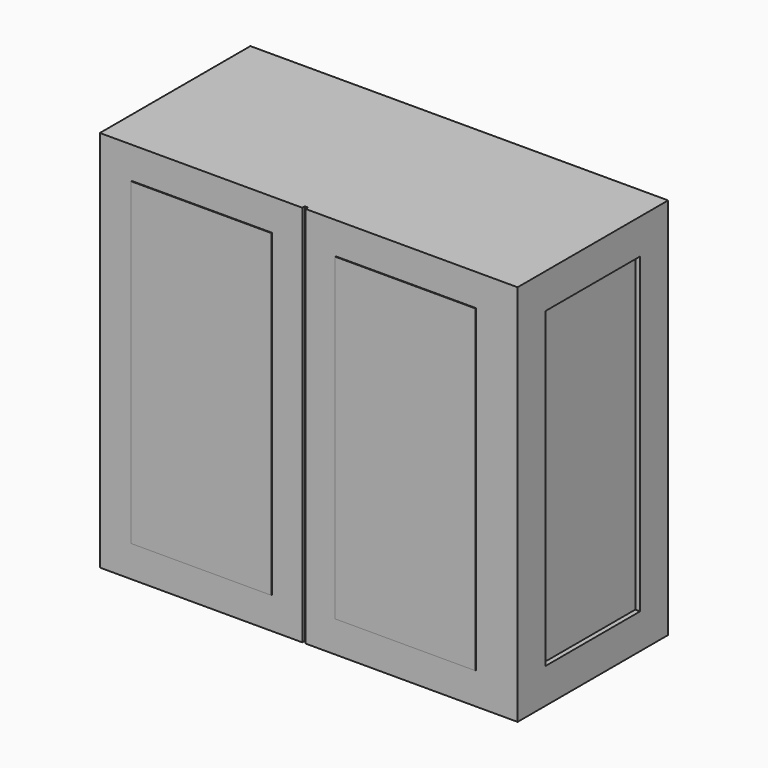
from build123d import *

# Parameters (mm, degrees)
F0_W     = 279.4
F0_H     = 635
F0_W_2   = 3.175
F0_H_2   = 762
F1_DEPTH = 374.65
F2_DEPTH = 6.35
F3_DEPTH = 1.524
F4_W     = 374.65
F4_H     = 762
F4_W_2   = 234.95
F4_H_2   = 622.3
F5_DEPTH = 19.05
F6_DEPTH = 9.525


# Not quite as in the source:
# - a feature names something its author has since deleted; it is built from what else it names


with BuildPart() as f1:
    # F0 (on Front) → F1 (new body)
    with BuildSketch(Plane.XZ):
        Polygon((-178.4927574873, 0), (224.7322425127, 0), (224.7322425127, 762), (151.7072425127, 762), (-178.4927574873, 762), align=None)
        with Locations((24.7072425127, 381)):
            Rectangle(F0_W, F0_H, mode=Mode.SUBTRACT)
        Polygon((231.0822425127, 762), (231.0822425127, 0), (634.3072425127, 0), (634.3072425127, 762), (304.1072425127, 762), align=None)
        with Locations((431.1072425127, 381)):
            Rectangle(F0_W, F0_H, mode=Mode.SUBTRACT)
        with Locations((24.7072425127, 381)):
            Rectangle(F0_W, F0_H)
        with Locations((431.1072425127, 381)):
            Rectangle(F0_W, F0_H)
        with Locations((226.3197425127, 381)):
            Rectangle(F0_W_2, F0_H_2)
        with Locations((229.4947425127, 381)):
            Rectangle(F0_W_2, F0_H_2)
    extrude(amount=-F1_DEPTH)

    # F0 (on Front) → F2 (cut)
    with BuildSketch(Plane.XZ):
        with Locations((226.3197425127, 381)):
            Rectangle(F0_W_2, F0_H_2)
        with Locations((229.4947425127, 381)):
            Rectangle(F0_W_2, F0_H_2)
        with Locations((24.7072425127, 381)):
            Rectangle(F0_W, F0_H)
        with Locations((431.1072425127, 381)):
            Rectangle(F0_W, F0_H)
    extrude(amount=-F2_DEPTH, mode=Mode.SUBTRACT)

    # F4 (on face) → F5 (join)
    with BuildSketch(Plane.YZ.offset(634.3072425127)):
        with Locations((187.325, 381)):
            Rectangle(F4_W, F4_H)
        with Locations((187.325, 381)):
            Rectangle(F4_W_2, F4_H_2, mode=Mode.SUBTRACT)
    extrude(amount=F5_DEPTH)

    # F6 (add): a face of the model
    f6_faces = [f1.faces().sort_by_distance(p)[0] for p in [
        (634.3072425127, 187.325, 381),
    ]]
    extrude(f6_faces, amount=F6_DEPTH)


with BuildPart() as f3:
    # F0 (on Front) → F3 (new body)
    with BuildSketch(Plane.XZ):
        with Locations((24.7072425127, 381)):
            Rectangle(F0_W, F0_H)
    extrude(amount=F3_DEPTH)


with BuildPart() as f3b:
    # F0 (on Front) → F3, piece 2 (new body)
    with BuildSketch(Plane.XZ):
        with Locations((431.1072425127, 381)):
            Rectangle(F0_W, F0_H)
    extrude(amount=F3_DEPTH)


solid = Compound([f1.part, f3.part, f3b.part])
